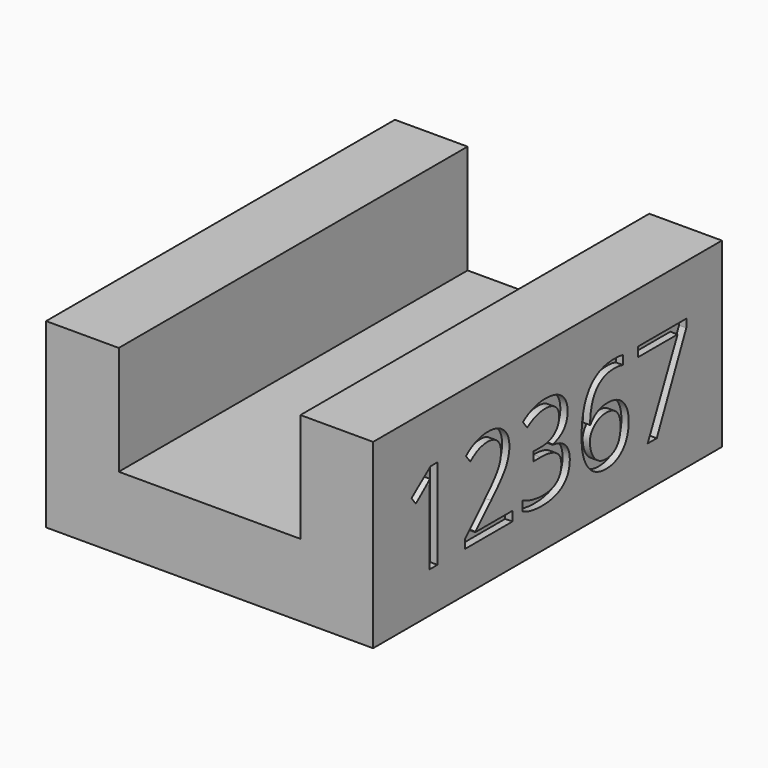
from build123d import *

# Parameters (mm, degrees)
F1_DEPTH     = 60
F2_TEXT_SIZE = 17.4054936089
F3_DEPTH     = 1


# Not quite as in the source:
# - Text() gives the source's letters only with a copy of the font that has no kerning and outlines rounded to 1/6400 em; it was checked with that copy


with BuildPart() as f1:
    # F0 (on Front) → F1 (new body)
    with BuildSketch(Plane.XZ):
        Polygon((-22.5, -10), (22.5, -10), (22.5, 15), (12.5, 15), (12.5, 0), (-12.5, 0), (-12.5, 15), (-22.5, 15), align=None)
    extrude(amount=F1_DEPTH)

    # F2 (on face) → F3 (cut)
    with BuildSketch(Plane.YZ.offset(22.5)):
        with Locations((-55, -4.3943218706)):
            Text('12367', F2_TEXT_SIZE, font='Open Sans', text_align=(TextAlign.LEFT, TextAlign.BOTTOM))
    extrude(amount=-F3_DEPTH, mode=Mode.SUBTRACT)


solid = f1.part
